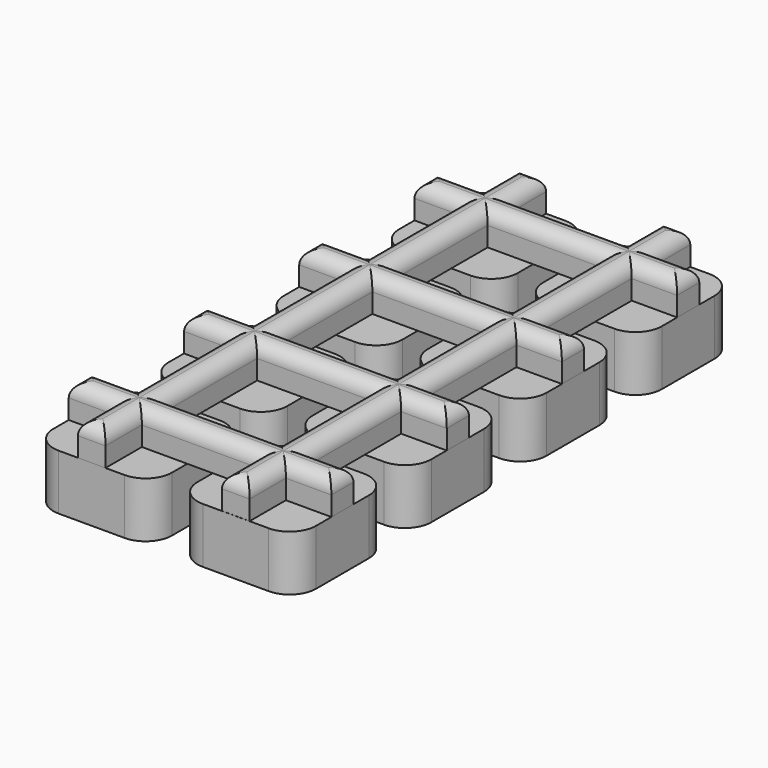
from build123d import *

# Parameters (mm, degrees)
F0_W     = 21.4
F0_H     = 21.4
F1_DEPTH = 10
F2_W     = 21
F2_H     = 21
F3_DEPTH = 6
F4_R     = 4.75
F4_2_R   = 4.75
F4_3_R   = 4.75
F4_4_R   = 4.75
F4_5_R   = 4.75
F4_6_R   = 4.75
F4_7_R   = 4.75
F4_8_R   = 4.75
F5_R     = 2.49999


# Not quite as in the source:
# - a fillet or chamfer is up to 0.001 mm smaller than in the source, because OpenCascade refuses the exact size


with BuildPart() as f1:
    # F0 (on Top) → F1 (new body)
    with BuildSketch(Plane.XY):
        Rectangle(F0_W, F0_H)
    extrude(amount=F1_DEPTH)

    # F4#8
    f4_8_edges = [f1.edges().sort_by_distance(p)[0] for p in [
        (10.7, -10.7, 5),
        (10.7, 10.7, 5),
        (-10.7, 10.7, 5),
        (-10.7, -10.7, 5),
    ]]
    fillet(f4_8_edges, radius=F4_8_R)


with BuildPart() as f1b:
    # F0 (on Top) → F1, piece 2 (new body)
    with BuildSketch(Plane.XY):
        with Locations((26, 0)):
            Rectangle(F0_W, F0_H)
    extrude(amount=F1_DEPTH)

    # F4#5
    f4_5_edges = [f1b.edges().sort_by_distance(p)[0] for p in [
        (36.7, -10.7, 5),
        (36.7, 10.7, 5),
        (15.3, -10.7, 5),
        (15.3, 10.7, 5),
    ]]
    fillet(f4_5_edges, radius=F4_5_R)


with BuildPart() as f1c:
    # F0 (on Top) → F1, piece 3 (new body)
    with BuildSketch(Plane.XY):
        with Locations((0, -26)):
            Rectangle(F0_W, F0_H)
    extrude(amount=F1_DEPTH)

    # F4#7
    f4_7_edges = [f1c.edges().sort_by_distance(p)[0] for p in [
        (10.7, -36.7, 5),
        (10.7, -15.3, 5),
        (-10.7, -15.3, 5),
        (-10.7, -36.7, 5),
    ]]
    fillet(f4_7_edges, radius=F4_7_R)


with BuildPart() as f1d:
    # F0 (on Top) → F1, piece 4 (new body)
    with BuildSketch(Plane.XY):
        with Locations((26, -26)):
            Rectangle(F0_W, F0_H)
    extrude(amount=F1_DEPTH)

    # F4#4
    f4_4_edges = [f1d.edges().sort_by_distance(p)[0] for p in [
        (36.7, -36.7, 5),
        (36.7, -15.3, 5),
        (15.3, -36.7, 5),
        (15.3, -15.3, 5),
    ]]
    fillet(f4_4_edges, radius=F4_4_R)


with BuildPart() as f1e:
    # F0 (on Top) → F1, piece 5 (new body)
    with BuildSketch(Plane.XY):
        with Locations((0, -52)):
            Rectangle(F0_W, F0_H)
    extrude(amount=F1_DEPTH)

    # F4#6
    f4_6_edges = [f1e.edges().sort_by_distance(p)[0] for p in [
        (10.7, -62.7, 5),
        (-10.7, -41.3, 5),
        (-10.7, -62.7, 5),
        (10.7, -41.3, 5),
    ]]
    fillet(f4_6_edges, radius=F4_6_R)


with BuildPart() as f1f:
    # F0 (on Top) → F1, piece 6 (new body)
    with BuildSketch(Plane.XY):
        with Locations((26, -52)):
            Rectangle(F0_W, F0_H)
    extrude(amount=F1_DEPTH)

    # F4#3
    f4_3_edges = [f1f.edges().sort_by_distance(p)[0] for p in [
        (36.7, -62.7, 5),
        (36.7, -41.3, 5),
        (15.3, -62.7, 5),
        (15.3, -41.3, 5),
    ]]
    fillet(f4_3_edges, radius=F4_3_R)


with BuildPart() as f1g:
    # F0 (on Top) → F1, piece 7 (new body)
    with BuildSketch(Plane.XY):
        with Locations((0, -78)):
            Rectangle(F0_W, F0_H)
    extrude(amount=F1_DEPTH)

    # F4#2
    f4_2_edges = [f1g.edges().sort_by_distance(p)[0] for p in [
        (10.7, -88.7, 5),
        (-10.7, -88.7, 5),
        (-10.7, -67.3, 5),
        (10.7, -67.3, 5),
    ]]
    fillet(f4_2_edges, radius=F4_2_R)


with BuildPart() as f1h:
    # F0 (on Top) → F1, piece 8 (new body)
    with BuildSketch(Plane.XY):
        with Locations((26, -78)):
            Rectangle(F0_W, F0_H)
    extrude(amount=F1_DEPTH)

    # F4
    f4_edges = [f1h.edges().sort_by_distance(p)[0] for p in [
        (36.7, -88.7, 5),
        (15.3, -88.7, 5),
        (36.7, -67.3, 5),
        (15.3, -67.3, 5),
    ]]
    fillet(f4_edges, radius=F4_R)


with BuildPart() as f3:
    # F2 (on face) → F3 (new body)
    with BuildSketch(Plane.XY.offset(10)):
        Polygon((-2.5, 2.5), (-10.7, 2.5), (-10.7, -2.5), (-2.5, -2.5), (-2.5, -23.5), (-10.7, -23.5), (-10.7, -28.5), (-2.5, -28.5), (-2.5, -49.5), (-10.6740258634, -49.5), (-10.6740258634, -54.5), (-2.5, -54.5), (-2.5, -75.5), (-10.7, -75.5), (-10.7, -80.5), (-2.5, -80.5), (-2.5, -88.7), (2.5, -88.7), (2.5, -80.5), (23.5, -80.5), (23.5, -88.6802822351), (28.5, -88.6802822351), (28.5, -80.5), (36.7, -80.5), (36.7, -75.5), (28.5, -75.5), (28.5, -54.5), (36.7259741366, -54.5), (36.7259741366, -49.5), (28.5, -49.5), (28.5, -28.5), (36.7, -28.5), (36.7, -23.5), (28.5, -23.5), (28.5, -2.5), (36.7, -2.5), (36.7, 2.5), (28.5, 2.5), (28.5, 10.7197177649), (23.5, 10.7197177649), (23.5, 2.5), (2.5, 2.5), (2.5, 10.7), (-2.5, 10.7), align=None)
        with Locations((13, -65)):
            Rectangle(F2_W, F2_H, mode=Mode.SUBTRACT)
        with Locations((13, -39)):
            Rectangle(F2_W, F2_H, mode=Mode.SUBTRACT)
        with Locations((13, -13)):
            Rectangle(F2_W, F2_H, mode=Mode.SUBTRACT)
    extrude(amount=F3_DEPTH)

    # F5 (radius 2.5 in the source; OpenCascade refuses exactly that, so slightly less here)
    f5_edges = [f3.edges().sort_by_distance(p)[0] for p in [
        (13, 2.5, 16),
        (26, 10.719718, 16),
        (23.5, 6.609859, 16),
        (0, 10.7, 16),
        (-6.6, -23.5, 16),
        (-2.5, 6.6, 16),
        (2.5, 6.6, 16),
        (-6.6, 2.5, 16),
        (28.5, 6.609859, 16),
        (32.6, 2.5, 16),
        (36.7, 0, 16),
        (-10.7, 0, 16),
        (-6.6, -2.5, 16),
        (-2.5, -13, 16),
        (-10.7, -26, 16),
        (-6.6, -28.5, 16),
        (-10.674026, -52, 16),
        (-6.587013, -49.5, 16),
        (-2.5, -39, 16),
        (2.5, -39, 16),
        (13, -28.5, 16),
        (-6.587013, -54.5, 16),
        (-2.5, -65, 16),
        (-6.6, -75.5, 16),
        (-10.7, -78, 16),
        (-6.6, -80.5, 16),
        (-2.5, -84.6, 16),
        (0, -88.7, 16),
        (2.5, -84.6, 16),
        (13, -80.5, 16),
        (23.5, -84.590141, 16),
        (26, -88.680282, 16),
        (28.5, -84.590141, 16),
        (32.6, -80.5, 16),
        (36.7, -78, 16),
        (32.6, -75.5, 16),
        (28.5, -65, 16),
        (32.612987, -54.5, 16),
        (36.725974, -52, 16),
        (32.612987, -49.5, 16),
        (28.5, -39, 16),
        (32.6, -28.5, 16),
        (36.7, -26, 16),
        (32.6, -23.5, 16),
        (28.5, -13, 16),
        (32.6, -2.5, 16),
        (13, -54.5, 16),
        (23.5, -65, 16),
        (13, -75.5, 16),
        (2.5, -65, 16),
        (23.5, -39, 16),
        (13, -49.5, 16),
        (13, -23.5, 16),
        (2.5, -13, 16),
        (13, -2.5, 16),
        (23.5, -13, 16),
    ]]
    fillet(f5_edges, radius=F5_R)


solid = Compound([f1.part, f1b.part, f1c.part, f1d.part, f1e.part, f1f.part, f1g.part, f1h.part, f3.part])
